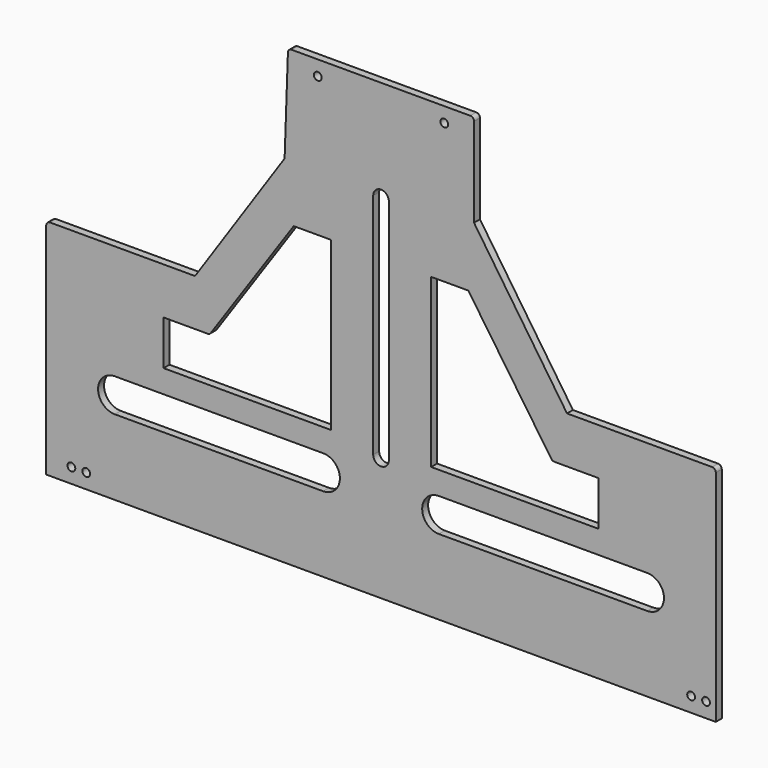
from build123d import *

# Parameters (mm, degrees)
F0_R     = 5.25
F1_DEPTH = 10
F2_R     = 5
F3_R     = 5


# Not quite as in the source:
# - ends of sketch curves that miss each other by under 0.0002 mm in the source are joined


with BuildPart() as f1:
    # F0 (on Front) → F1 (new body)
    with BuildSketch(Plane.XZ):
        Polygon((-250, 62.7604842186), (-450, 62.7604842186), (-450, -237.2395157814), (0, -237.2395157814), (450, -237.2395157814), (450, 62.7604842186), (250, 62.7604842186), (125, 247.7604842186), (125, 372.7604842186), (-125, 372.7604842186), (-129.5981111256, 240.9552797528), align=None)
        with Locations((-416.2039160728, -217.2395157814)):
            Circle(F0_R, mode=Mode.SUBTRACT)
        with Locations((-396.2039160728, -217.2395157814)):
            Circle(F0_R, mode=Mode.SUBTRACT)
        with BuildLine():
            Line((-357.8152358532, -90.9260827303), (-77.8152358532, -90.9260827303))
            ThreePointArc((-77.8152358532, -90.9260827303), (-55.3152358532, -113.4260827303), (-77.8152358532, -135.9260827303))
            Line((-77.8152358532, -135.9260827303), (-357.8152358532, -135.9260827303))
            ThreePointArc((-357.8152358532, -135.9260827303), (-380.3152358532, -113.4260827303), (-357.8152358532, -90.9260827303))
        make_face(mode=Mode.SUBTRACT)
        Polygon((-292.343990892, -60), (-292.343990892, 0), (-230.3705364466, 0), (-117.343990892, 165), (-67.343990892, 165), (-67.343990892, 0), (-67.343990892, -60), align=None, mode=Mode.SUBTRACT)
        with BuildLine():
            ThreePointArc((77.8152358532, -135.9260827303), (55.3152358532, -113.4260827303), (77.8152358532, -90.9260827303))
            Line((77.8152358532, -90.9260827303), (357.8152358532, -90.9260827303))
            ThreePointArc((357.8152358532, -90.9260827303), (380.3152358532, -113.4260827303), (357.8152358532, -135.9260827303))
            Line((357.8152358532, -135.9260827303), (77.8152358532, -135.9260827303))
        make_face(mode=Mode.SUBTRACT)
        with Locations((416.8414473534, -217.2395157814)):
            Circle(F0_R, mode=Mode.SUBTRACT)
        with Locations((436.8414473534, -217.2395157814)):
            Circle(F0_R, mode=Mode.SUBTRACT)
        Polygon((67.343990892, 0), (67.343990892, 165), (117.343990892, 165), (230.3705364466, 0), (292.343990892, 0), (292.343990892, -60), (67.343990892, -60), align=None, mode=Mode.SUBTRACT)
        with Locations((-85, 352.7604842186)):
            Circle(F0_R, mode=Mode.SUBTRACT)
        with BuildLine():
            Line((-10.5, 235.874648428), (-10.5, 235.897347331))
            ThreePointArc((-10.5, 235.897347331), (0.0113494317, 246.3746422942), (10.5, 235.874648428))
            Line((10.5, 235.874648428), (10.5, 0.0226989031))
            Line((10.5, 0.0226989031), (10.5, -70.725351572))
            ThreePointArc((10.5, -70.725351572), (0, -81.225351572), (-10.5, -70.725351572))
            Line((-10.5, -70.725351572), (-10.5, 0))
            Line((-10.5, 0), (-10.5, 235.874648428))
        make_face(mode=Mode.SUBTRACT)
        with Locations((85, 352.7604842186)):
            Circle(F0_R, mode=Mode.SUBTRACT)
    extrude(amount=F1_DEPTH)

    # F2
    f2_edges = [f1.edges().sort_by_distance(p)[0] for p in [
        (-230.370536, -5, 0),
        (230.370536, -5, 0),
    ]]
    fillet(f2_edges, radius=F2_R)

    # F3
    f3_edges = [f1.edges().sort_by_distance(p)[0] for p in [
        (-450, -5, 62.760484),
        (-125, -5, 372.760484),
        (125, -5, 372.760484),
        (450, -5, 62.760484),
    ]]
    fillet(f3_edges, radius=F3_R)


solid = f1.part
